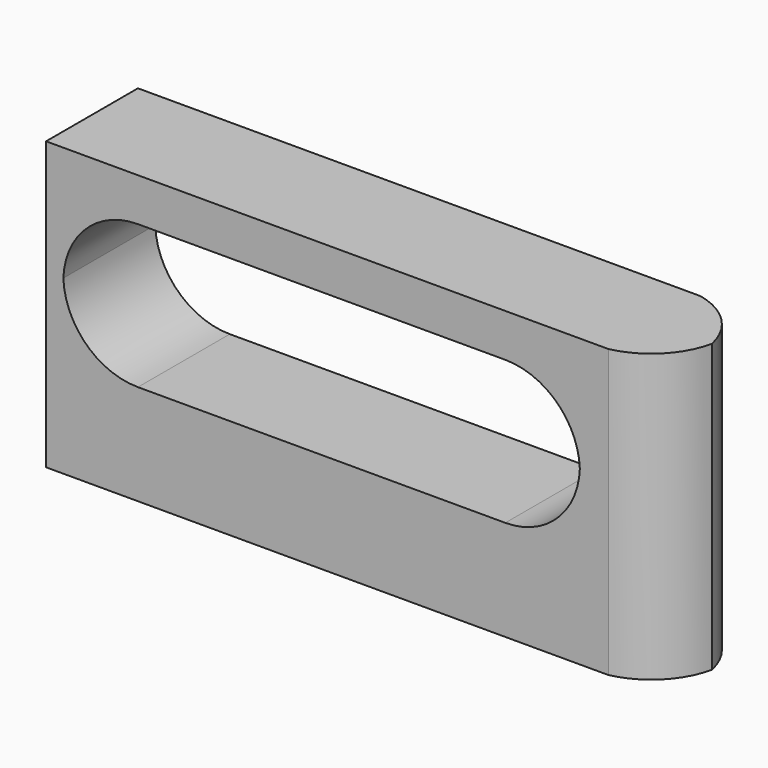
from build123d import *

# Parameters (mm, degrees)
F1_DEPTH    = 5
F2_W        = 9
F2_H        = 2.5
F3_DEPTH    = 2.001
F4_T1_DEPTH = 2
F6_DEPTH    = 5.001


# Not quite as in the source:
# - a fillet or chamfer that OpenCascade refuses, or shapes differently, is made with other operations: its cross-section is extruded or revolved along the edge and cut away or added


with BuildPart() as f1:
    # F0 (on Top) → F1 (new body)
    with BuildSketch(Plane.XY):
        with BuildLine():
            Line((5, 1), (-5, 1))
            ThreePointArc((-5, 1), (-5.6464466094, 0.6464466094), (-6, 0))
            ThreePointArc((-6, 0), (-5.6464466094, -0.6464466094), (-5, -1))
            Line((-5, -1), (5, -1))
            ThreePointArc((5, -1), (5.6464466094, -0.6464466094), (6, 0))
            ThreePointArc((6, 0), (5.6464466094, 0.6464466094), (5, 1))
        make_face()
    extrude(amount=F1_DEPTH)

    # F2 (on face) → F3 (cut, through all)
    with BuildSketch(Plane.XZ.offset(1)):
        with Locations((0, 3)):
            Rectangle(F2_W, F2_H)
    extrude(amount=-F3_DEPTH, mode=Mode.SUBTRACT)

    # F4: fillet of radius 1.3 on 4 edges, made by hand

    # F4_s2 → F4_t1 (join)
    with BuildSketch(Plane.XZ.offset(-1)):
        with BuildLine():
            ThreePointArc((-4.5, 3.05), (-4.1192388155, 2.1307611845), (-3.2, 1.75))
            Line((-3.2, 1.75), (-4.5, 1.75))
            Line((-4.5, 1.75), (-4.5, 3.05))
        make_face()
        with BuildLine():
            ThreePointArc((-3.2, 4.25), (-4.1192388155, 3.8692388155), (-4.5, 2.95))
            Line((-4.5, 2.95), (-4.5, 4.25))
            Line((-4.5, 4.25), (-3.2, 4.25))
        make_face()
        with BuildLine():
            ThreePointArc((3.2, 4.25), (4.1192388155, 3.8692388155), (4.5, 2.95))
            Line((4.5, 2.95), (4.5, 4.25))
            Line((4.5, 4.25), (3.2, 4.25))
        make_face()
        with BuildLine():
            ThreePointArc((3.2, 1.75), (4.1192388155, 2.1307611845), (4.5, 3.05))
            Line((4.5, 3.05), (4.5, 1.75))
            Line((4.5, 1.75), (3.2, 1.75))
        make_face()
    extrude(amount=F4_T1_DEPTH)

    # F5 (on face) → F6 (cut, through all)
    with BuildSketch(Plane.XY.offset(5)):
        with BuildLine():
            Line((-4.8, -1), (-4.8, 1))
            Line((-4.8, 1), (-5, 1))
            ThreePointArc((-5, 1), (-5.6464466094, 0.6464466094), (-6, 0))
            ThreePointArc((-6, 0), (-5.6464466094, -0.6464466094), (-5, -1))
            Line((-5, -1), (-4.8, -1))
        make_face()
    extrude(amount=-F6_DEPTH, mode=Mode.SUBTRACT)


solid = f1.part
